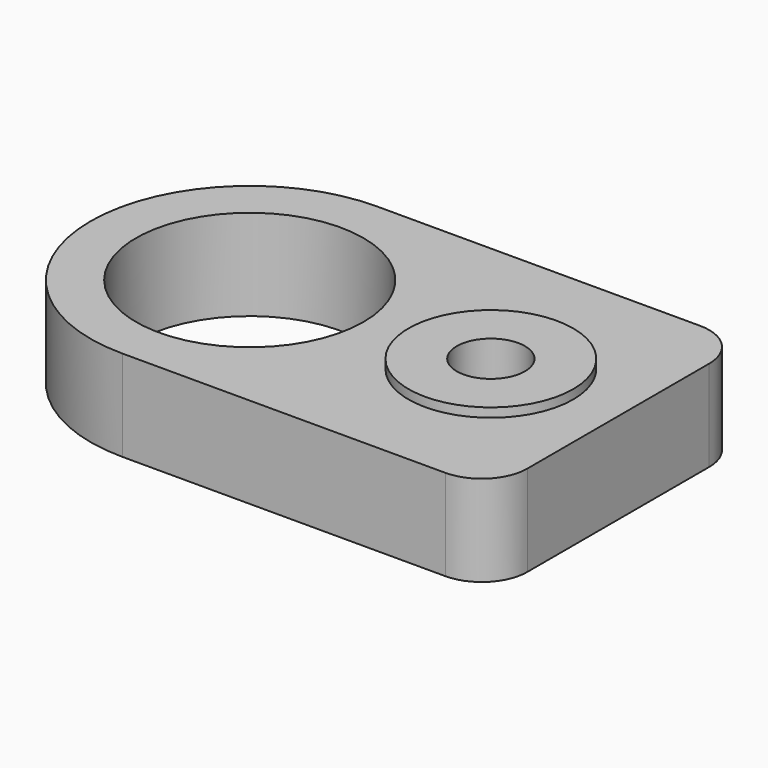
from build123d import *

# Parameters (mm, degrees)
F0_R         = 12.5
F1_DEPTH     = 10
F2_R         = 9.05
F2_R_2       = 3.75
F3_DEPTH     = 1
F4_DEPTH     = 7.5
F5_TEXT_SIZE = 5.5555555556
F6_DEPTH     = 1


# Not quite as in the source:
# - Text() gives the source's letters only with a copy of the font that has no kerning and outlines rounded to 1/6400 em; it was checked with that copy


with BuildPart() as f1:
    # F0 (on Top) → F1 (new body)
    with BuildSketch(Plane.XY):
        with BuildLine():
            ThreePointArc((0, 17.5), (5.1256313292, 5.1256313292), (17.5, 0))
            Line((17.5, 0), (53, 0))
            ThreePointArc((53, 0), (56.5355339059, 1.4644660941), (58, 5))
            Line((58, 5), (58, 30))
            ThreePointArc((58, 30), (56.5355339059, 33.5355339059), (53, 35))
            Line((53, 35), (17.5, 35))
            ThreePointArc((17.5, 35), (5.1256313292, 29.8743686708), (0, 17.5))
        make_face()
        with Locations((17.5, 17.5)):
            Circle(F0_R, mode=Mode.SUBTRACT)
    extrude(amount=F1_DEPTH)

    # F2 (on face) → F3 (join)
    with BuildSketch(Plane.XY.offset(10)):
        with Locations((44, 17.5)):
            Circle(F2_R)
        with Locations((44, 17.5)):
            Circle(F2_R_2, mode=Mode.SUBTRACT)
    extrude(amount=F3_DEPTH)

    # F2 (on face) → F4 (cut)
    with BuildSketch(Plane.XY.offset(10)):
        with Locations((44, 17.5)):
            Circle(F2_R_2)
    extrude(amount=-F4_DEPTH, mode=Mode.SUBTRACT)

    # F5 (on face) → F6 (cut)
    with BuildSketch(Plane(origin=(0, 0, 0), x_dir=(1, 0, 0), z_dir=(0, 0, -1))):
        with Locations((30, -9)):
            Text('854', F5_TEXT_SIZE, font='Open Sans', text_align=(TextAlign.LEFT, TextAlign.BOTTOM))
    extrude(amount=-F6_DEPTH, mode=Mode.SUBTRACT)


solid = f1.part
